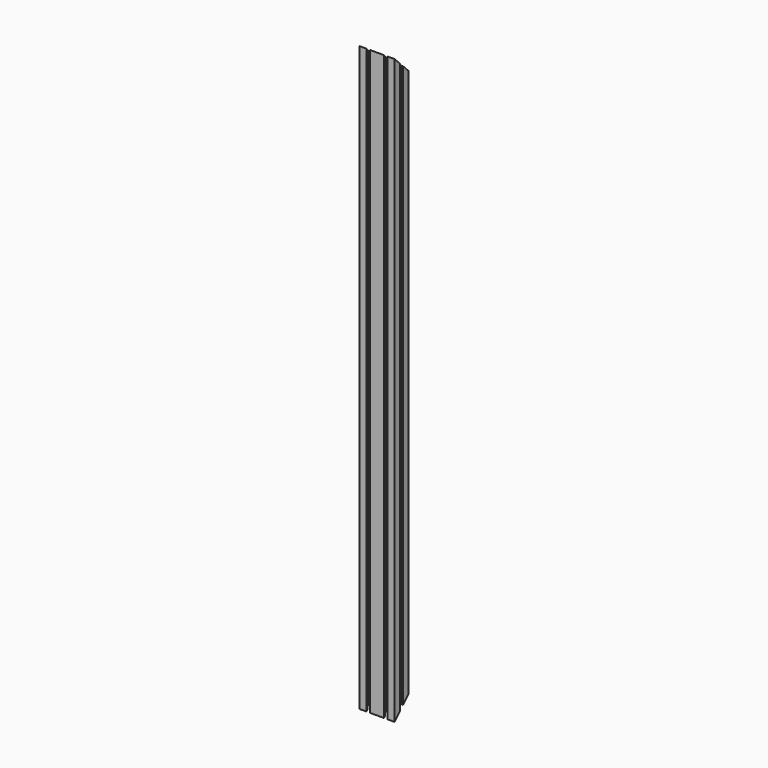
from build123d import *

# Parameters (mm, degrees)
F0_R     = 3
F0_R_2   = 2.5
F1_DEPTH = 1000
F2_R     = 2
F3_R     = 7
F5_DEPTH = 30


# Not quite as in the source:
# - a feature names something its author has since deleted; it is built from what else it names


with BuildPart() as f1:
    # F0 (on Top) → F1 (new body)
    with BuildSketch(Plane.XY):
        with BuildLine():
            Line((18.15, -15), (30, -15))
            Line((30, -15), (30, -3.15))
            Line((30, -3.15), (27.5, -3.15))
            Line((27.5, -3.15), (27.5, -5.15))
            Line((27.5, -5.15), (21.5477069044, -5.15))
            ThreePointArc((21.5477069044, -5.15), (19.5, 0), (21.5477069044, 5.15))
            Line((21.5477069044, 5.15), (27.5, 5.15))
            Line((27.5, 5.15), (27.5, 3.15))
            Line((27.5, 3.15), (30, 3.15))
            Line((30, 3.15), (30, 15))
            Line((30, 15), (18.15, 15))
            Line((18.15, 15), (18.15, 12.5))
            Line((18.15, 12.5), (20.15, 12.5))
            Line((20.15, 12.5), (20.15, 6.5477069044))
            ThreePointArc((20.15, 6.5477069044), (15, 4.5), (9.85, 6.5477069044))
            Line((9.85, 6.5477069044), (9.85, 12.5))
            Line((9.85, 12.5), (11.85, 12.5))
            Line((11.85, 12.5), (11.85, 15))
            Line((11.85, 15), (-11.85, 15))
            Line((-11.85, 15), (-11.85, 12.5))
            Line((-11.85, 12.5), (-9.85, 12.5))
            Line((-9.85, 12.5), (-9.85, 6.5477069044))
            ThreePointArc((-9.85, 6.5477069044), (-15, 4.5), (-20.15, 6.5477069044))
            Line((-20.15, 6.5477069044), (-20.15, 12.5))
            Line((-20.15, 12.5), (-18.15, 12.5))
            Line((-18.15, 12.5), (-18.15, 15))
            Line((-18.15, 15), (-30, 15))
            Line((-30, 15), (-30, 3.15))
            Line((-30, 3.15), (-27.5, 3.15))
            Line((-27.5, 3.15), (-27.5, 5.15))
            Line((-27.5, 5.15), (-21.5477069044, 5.15))
            ThreePointArc((-21.5477069044, 5.15), (-19.5, 0), (-21.5477069044, -5.15))
            Line((-21.5477069044, -5.15), (-27.5, -5.15))
            Line((-27.5, -5.15), (-27.5, -3.15))
            Line((-27.5, -3.15), (-30, -3.15))
            Line((-30, -3.15), (-30, -15))
            Line((-30, -15), (-18.15, -15))
            Line((-18.15, -15), (-18.15, -12.5))
            Line((-18.15, -12.5), (-20.15, -12.5))
            Line((-20.15, -12.5), (-20.15, -6.5477069044))
            ThreePointArc((-20.15, -6.5477069044), (-15, -4.5), (-9.85, -6.5477069044))
            Line((-9.85, -6.5477069044), (-9.85, -12.5))
            Line((-9.85, -12.5), (-11.85, -12.5))
            Line((-11.85, -12.5), (-11.85, -15))
            Line((-11.85, -15), (11.85, -15))
            Line((11.85, -15), (11.85, -12.5))
            Line((11.85, -12.5), (9.85, -12.5))
            Line((9.85, -12.5), (9.85, -6.5477069044))
            ThreePointArc((9.85, -6.5477069044), (15, -4.5), (20.15, -6.5477069044))
            Line((20.15, -6.5477069044), (20.15, -12.5))
            Line((20.15, -12.5), (18.15, -12.5))
            Line((18.15, -12.5), (18.15, -15))
        make_face()
        with Locations((-25, -10)):
            Circle(F0_R, mode=Mode.SUBTRACT)
        with Locations((25, -10)):
            Circle(F0_R, mode=Mode.SUBTRACT)
        with Locations((-15, 0)):
            Circle(F0_R_2, mode=Mode.SUBTRACT)
        with Locations((-25, 10)):
            Circle(F0_R, mode=Mode.SUBTRACT)
        Polygon((-7, 7), (-7, 12.5), (0, 12.5), (7, 12.5), (7, 7), (10, 0), (7, -7), (7, -12.5), (0, -12.5), (-7, -12.5), (-7, -7), (-10, 0), align=None, mode=Mode.SUBTRACT)
        with Locations((15, 0)):
            Circle(F0_R_2, mode=Mode.SUBTRACT)
        with Locations((25, 10)):
            Circle(F0_R, mode=Mode.SUBTRACT)
    extrude(amount=F1_DEPTH)

    # F2
    f2_edges = [f1.edges().sort_by_distance(p)[0] for p in [
        (-7, 12.5, 500),
        (7, 12.5, 500),
    ]]
    fillet(f2_edges, radius=F2_R)

    # F3
    f3_edges = [f1.edges().sort_by_distance(p)[0] for p in [
        (-7, 7, 500),
        (-10, 0, 500),
        (7, 7, 500),
        (10, 0, 500),
    ]]
    fillet(f3_edges, radius=F3_R)

    # F4 (on Right) → F5 (cut, symmetric)
    with BuildSketch(Plane.YZ):
        Polygon((15, 30), (-15, 0), (15, 0), align=None)
        Polygon((15, 1000), (-15, 1000), (15, 970), align=None)
    extrude(amount=F5_DEPTH, both=True, mode=Mode.SUBTRACT)


solid = f1.part
